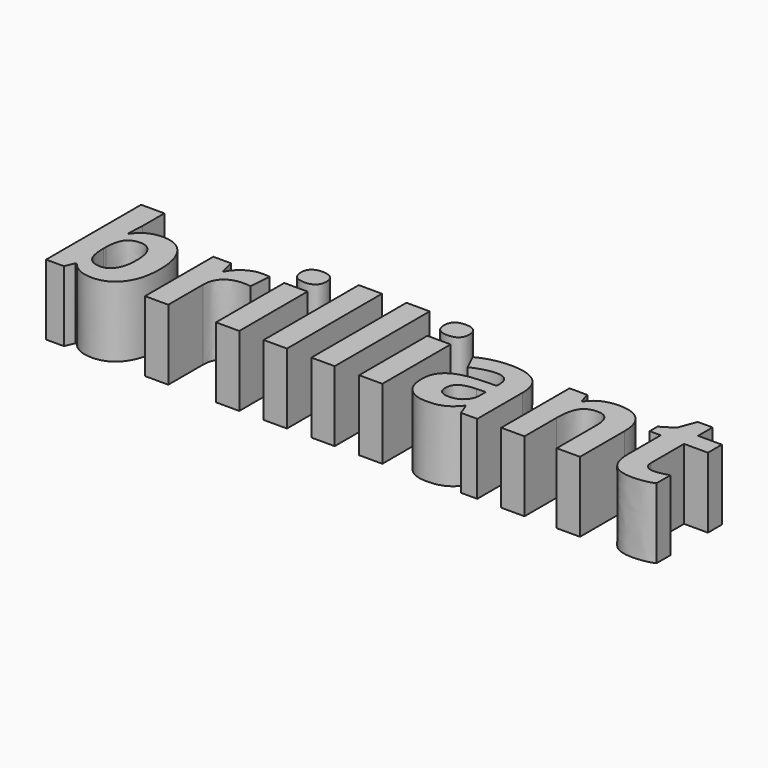
from build123d import *

# Parameters (mm, degrees)
F0_TEXT_SIZE = 56.3793194791
F1_DEPTH     = 25.4


# Not quite as in the source:
# - Text() gives the source's letters only with a copy of the font that has no kerning and outlines rounded to 1/6400 em; it was checked with that copy


with BuildPart() as f1:
    # F0 (on Top) → F1 (new body)
    with BuildSketch(Plane.XY):
        with Locations((-52.0369186997, -24.6149711311)):
            Text('brilliant', F0_TEXT_SIZE, font='Open Sans', font_style=FontStyle.BOLD, text_align=(TextAlign.LEFT, TextAlign.BOTTOM))
    extrude(amount=F1_DEPTH)


solid = f1.part
